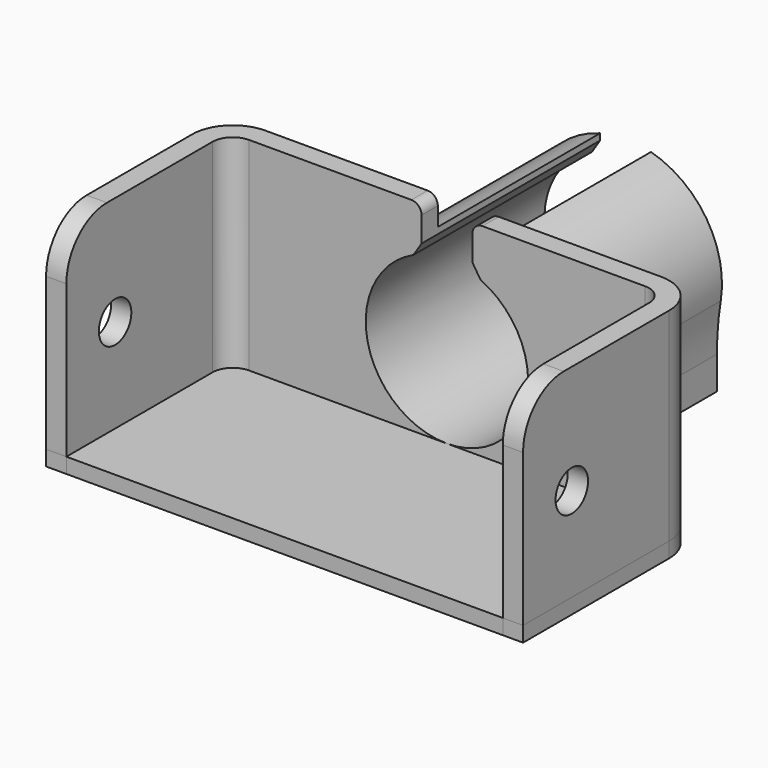
from build123d import *

# Parameters (mm, degrees)
F1_DEPTH     = 20
F2_R         = 2
F3_R         = 4
F5_DEPTH     = 1.5
F6_R         = 8
F7_DEPTH     = 20
F8_DEPTH     = 25
F9_W         = 5
F9_H         = 35.9879870677
F9_H_2       = 3.0384219572
F9_H_3       = 2
F10_DEPTH    = 12.4
F11_T1_DEPTH = 26.8776444438
F12_R        = 1
F13_R        = 5
F15_DEPTH    = 20
F17_DEPTH    = 20
F18_R        = 30
F19_R        = 2
F20_DEPTH    = 58


# Not quite as in the source:
# - a fillet or chamfer that OpenCascade refuses, or shapes differently, is made with other operations: its cross-section is extruded or revolved along the edge and cut away or added
# - ends of sketch curves that miss each other by under 0.0002 mm in the source are joined


with BuildPart() as f1:
    # F0 (on Top) → F1 (new body)
    with BuildSketch(Plane.XY):
        Polygon((-21.4999990134, 20), (21.5000009866, 20), (21.5, 0), (23.5, 0), (23.5000010853, 22), (-23.4999989147, 22), (-23.5, 0), (-21.5, 0), align=None)
    extrude(amount=F1_DEPTH)

    # F2
    f2_edges = [f1.edges().sort_by_distance(p)[0] for p in [
        (-21.499999, 20, 10),
        (21.500001, 20, 10),
    ]]
    fillet(f2_edges, radius=F2_R)

    # F3
    f3_edges = [f1.edges().sort_by_distance(p)[0] for p in [
        (-23.499999, 22, 10),
        (23.500001, 22, 10),
    ]]
    fillet(f3_edges, radius=F3_R)

    # F4 (on face) → F5 (join)
    with BuildSketch(Plane(origin=(0, 0, 0), x_dir=(1, 0, 0), z_dir=(0, 0, -1))):
        with BuildLine():
            Line((21.500000888, -17.9999999013), (21.5, 0))
            Line((21.5, 0), (-21.5, -2.2199e-06))
            Line((-21.5, -2.2199e-06), (-21.499999112, -18.0000000987))
            ThreePointArc((-21.499999112, -18.0000000987), (-20.9142126395, -19.4142135973), (-19.499999112, -20))
            Line((-19.499999112, -20), (19.500000888, -20))
            ThreePointArc((19.500000888, -20), (20.9142144852, -19.4142135275), (21.500000888, -17.9999999013))
        make_face()
        with BuildLine():
            ThreePointArc((19.500000888, -22), (22.3284280825, -20.828427055), (23.500000888, -17.9999998027))
            Line((23.500000888, -17.9999998027), (23.5, 0))
            Line((23.5, 0), (21.5, -9.87e-08))
            Line((21.5, -9.87e-08), (21.500000888, -17.9999999013))
            ThreePointArc((21.500000888, -17.9999999013), (20.9142144852, -19.4142135275), (19.500000888, -20))
            Line((19.500000888, -20), (-19.499999112, -20))
            ThreePointArc((-19.499999112, -20), (-20.9142126395, -19.4142135973), (-21.499999112, -18.0000000987))
            Line((-21.499999112, -18.0000000987), (-21.5, 0))
            Line((-21.5, 0), (-23.5, -2.3186e-06))
            Line((-23.5, -2.3186e-06), (-23.499999112, -18.0000001973))
            ThreePointArc((-23.499999112, -18.0000001973), (-22.328426167, -20.8284271945), (-19.499999112, -22))
            Line((-19.499999112, -22), (19.500000888, -22))
        make_face()
    extrude(amount=F5_DEPTH)

    # F6 (on face) → F7 (join)
    with BuildSketch(Plane(origin=(0, 22, 0), x_dir=(-1, 0, 0), z_dir=(0, 1, 0))):
        with BuildLine():
            ThreePointArc((4.21e-08, -1.5), (6.7175144362, 1.2824855936), (9.5, 8))
            ThreePointArc((9.5, 8), (-6.7175144362, 14.7175144064), (4.21e-08, -1.5))
        make_face()
        with Locations((0, 8)):
            Circle(F6_R, mode=Mode.SUBTRACT)
    extrude(amount=F7_DEPTH)

    # F8 (cut): a face of the model
    f8_faces = [f1.faces().sort_by_distance(p)[0] for p in [
        (0, 22, 8),
    ]]
    extrude(f8_faces, amount=-F8_DEPTH, mode=Mode.SUBTRACT)

    # F9 (on face) → F10 (cut)
    with BuildSketch(Plane.XY.offset(20)):
        with Locations((0, 39.9939935338)):
            Rectangle(F9_W, F9_H)
        with Locations((0, 18.4807890214)):
            Rectangle(F9_W, F9_H_2)
        with Locations((0, 21)):
            Rectangle(F9_W, F9_H_3)
    extrude(amount=-F10_DEPTH, mode=Mode.SUBTRACT)

    # F11: chamfer of 1 on 2 edges, made by hand

    # F11_s2 → F11_t1 (cut)
    with BuildSketch(Plane.XZ.offset(-44.4388222219)):
        with BuildLine():
            Line((-3.3316740869, 15.2494859065), (-2.4783436331, 16.5746305544))
            Line((-2.4783436331, 16.5746305544), (-2.4583436331, 16.5746305544))
            ThreePointArc((-2.4583436331, 16.5746305544), (-2.48, 16.0869863156), (-2.48, 15.5993420768))
            Line((-2.48, 15.5993420768), (-2.49375, 15.5803437216))
            ThreePointArc((-2.49375, 15.5803437216), (-2.9171284808, 15.4277022979), (-3.3233990426, 15.2312781158))
            Line((-3.3233990426, 15.2312781158), (-3.3316740869, 15.2494859065))
        make_face()
        with BuildLine():
            Line((2.4783436331, 16.5746305544), (3.3316740869, 15.2494859065))
            Line((3.3316740869, 15.2494859065), (3.3233990426, 15.2312781158))
            ThreePointArc((3.3233990426, 15.2312781158), (2.9171284808, 15.4277022979), (2.49375, 15.5803437216))
            Line((2.49375, 15.5803437216), (2.48, 15.5993420768))
            ThreePointArc((2.48, 15.5993420768), (2.48, 16.0869863156), (2.4583436331, 16.5746305544))
            Line((2.4583436331, 16.5746305544), (2.4783436331, 16.5746305544))
        make_face()
    extrude(amount=F11_T1_DEPTH, mode=Mode.SUBTRACT)

    # F12
    f12_edges = [f1.edges().sort_by_distance(p)[0] for p in [
        (2.5, 21, 20),
        (-2.5, 21, 20),
    ]]
    fillet(f12_edges, radius=F12_R)

    # F13
    f13_edges = [f1.edges().sort_by_distance(p)[0] for p in [
        (-22.5, 0, 20),
        (22.5, 0, 20),
    ]]
    fillet(f13_edges, radius=F13_R)

    # F14 (on face) → F15 (join)
    with BuildSketch(Plane(origin=(0, 22, 0), x_dir=(-1, 0, 0), z_dir=(0, 1, 0))):
        with BuildLine():
            ThreePointArc((2.1e-08, -1.5), (-5.5388120473, 0.2817384662), (-9, 4.9586187349))
            Line((-9, 4.9586187349), (-9, -1.5))
            Line((-9, -1.5), (0, -1.5))
        make_face()
        with BuildLine():
            ThreePointArc((9, 4.9586187349), (5.5388120644, 0.2817384785), (2.1e-08, -1.5))
            Line((0, -1.5), (9, -1.5))
            Line((9, -1.5), (9, 4.9586187349))
        make_face()
    extrude(amount=F15_DEPTH)

    # F16 (on face) → F17 (cut)
    with BuildSketch(Plane(origin=(0, 42, 0), x_dir=(-1, 0, 0), z_dir=(0, 1, 0))):
        with BuildLine():
            ThreePointArc((-7, 2.3431457505), (-7.53910447, 3.0845240526), (-8, 3.8768943744))
            Line((-8, 3.8768943744), (-8, -0.5))
            Line((-8, -0.5), (-7, -0.5))
            Line((-7, -0.5), (-7, 2.3431457505))
        make_face()
        with BuildLine():
            Line((8, -0.5), (8, 3.8768943744))
            ThreePointArc((8, 3.8768943744), (7.53910447, 3.0845240526), (7, 2.3431457505))
            Line((7, 2.3431457505), (7, -0.5))
            Line((7, -0.5), (8, -0.5))
        make_face()
        with BuildLine():
            ThreePointArc((-4.8538187839, 0.4210526316), (-5.4443451471, 0.8334732318), (-6, 1.2917960675))
            Line((-6, 1.2917960675), (-6, -0.5))
            Line((-6, -0.5), (-5.123475383, -0.5))
            ThreePointArc((-5.123475383, -0.5), (-4.643617948, -0.1404878717), (-4.8538187839, 0.4210526316))
        make_face()
        with BuildLine():
            Line((6, -0.5), (6, 1.2917960675))
            ThreePointArc((6, 1.2917960675), (5.4443451471, 0.8334732318), (4.8538187839, 0.4210526316))
            ThreePointArc((4.8538187839, 0.4210526316), (4.643617948, -0.1404878717), (5.123475383, -0.5))
            Line((5.123475383, -0.5), (6, -0.5))
        make_face()
    extrude(amount=-F17_DEPTH, mode=Mode.SUBTRACT)

    # F18
    f18_edges = [f1.edges().sort_by_distance(p)[0] for p in [
        (-9, 32, 4.958619),
        (9, 32, 4.958619),
    ]]
    fillet(f18_edges, radius=F18_R)

    # F19 (on face) → F20 (cut)
    with BuildSketch(Plane(origin=(-23.5, 1.1593e-06, 0), x_dir=(-4.93e-08, -1, 0), z_dir=(-1, 4.93e-08, 0))):
        with Locations((-5.999999038, 9.25)):
            Circle(F19_R)
    extrude(amount=-F20_DEPTH, mode=Mode.SUBTRACT)


solid = f1.part
